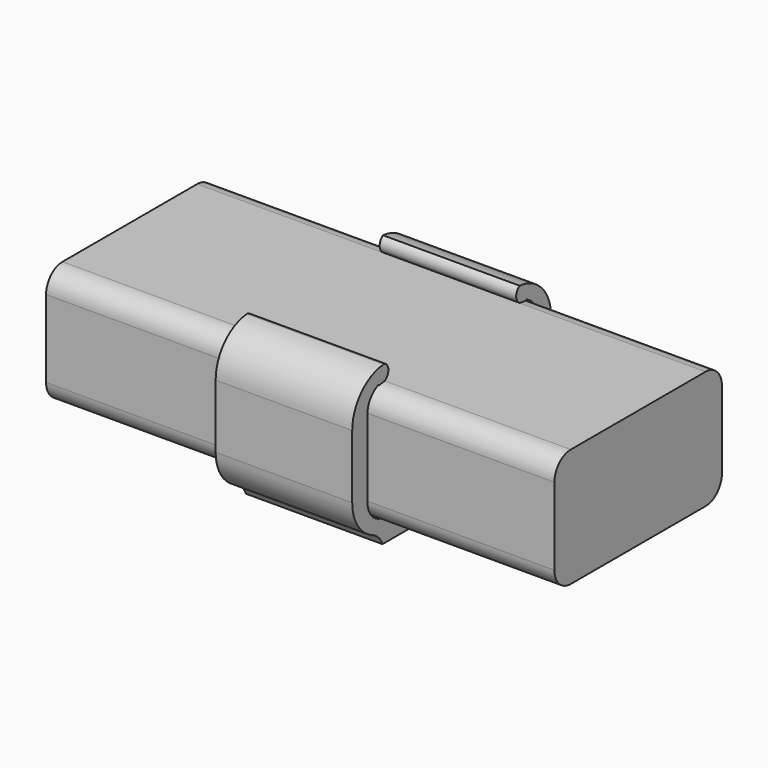
from build123d import *

# Parameters (mm, degrees)
F1_DEPTH       = 55.825
F3_DEPTH       = 15
F5_D           = 6.5
F5_CBORE_D     = 10.6
F5_CBORE_DEPTH = 3.4
F6_T1_DEPTH    = 30
F7_R           = 1


# Not quite as in the source:
# - a fillet or chamfer that OpenCascade refuses, or shapes differently, is made with other operations: its cross-section is extruded or revolved along the edge and cut away or added


with BuildPart() as f1:
    # F0 (on Right) → F1 (new body, symmetric)
    with BuildSketch(Plane.YZ):
        with BuildLine():
            ThreePointArc((-23, 4.5), (-21.6819805153, 1.3180194847), (-18.5, 0))
            Line((-18.5, 0), (18.5, 0))
            ThreePointArc((18.5, 0), (21.6819805153, 1.3180194847), (23, 4.5))
            Line((23, 4.5), (23, 21.5))
            ThreePointArc((23, 21.5), (21.6819805153, 24.6819805153), (18.5, 26))
            Line((18.5, 26), (-18.5, 26))
            ThreePointArc((-18.5, 26), (-21.6819805153, 24.6819805153), (-23, 21.5))
            Line((-23, 21.5), (-23, 4.5))
        make_face()
    extrude(amount=F1_DEPTH, both=True)


with BuildPart() as f3:
    # F2 (on Right) → F3 (new body, symmetric)
    with BuildSketch(Plane.YZ):
        with BuildLine():
            add(Edge.make_bspline(
                [(26.7413663264, 22.9510836938), (26.7479851877, 22.9405500746), (26.746124128, 22.9346023266), (26.7444516472, 22.9402163477)],
                knots=[0.9580519354, 0.9580519354, 0.9580519354, 0.9580519354, 1, 1, 1, 1], degree=3))
            ThreePointArc((26.7413663264, 22.9510836938), (26.7429106369, 22.9456504892), (26.7444516472, 22.9402163477))
        make_face()
    extrude(amount=F3_DEPTH, both=True)


with BuildPart() as f3b:
    # F2 (on Right) → F3, piece 2 (new body, symmetric)
    with BuildSketch(Plane.YZ):
        with BuildLine():
            Line((23.3, 21.5), (23.3, 4.5))
            ThreePointArc((23.3, 4.5), (21.8941125497, 1.1058874503), (18.5, -0.3))
            Line((18.5, -0.3), (-18.5, -0.3))
            ThreePointArc((-18.5, -0.3), (-21.8941125497, 1.1058874503), (-23.3, 4.5))
            Line((-23.3, 4.5), (-23.3, 21.5))
            ThreePointArc((-23.3, 21.5), (-22.4816132456, 24.1808125563), (-20.3055183491, 25.9474828264))
            ThreePointArc((-20.3055183491, 25.9474828264), (-17.7711928448, 26.7933262745), (-18.4856994576, 29.3677654758))
            ThreePointArc((-18.4856994576, 29.3677654758), (-24.8705621503, 26.5239553831), (-27.4715276401, 20.0363744805))
            Line((-27.4715276401, 20.0363744805), (-27.4715276401, 6.0863744805))
            ThreePointArc((-27.4715276401, 6.0863744805), (-25.0921489995, -0.126112944), (-19.1715276401, -3.1597057701))
            Line((-19.1715276401, -3.1597057701), (-19.1715276401, -5.3))
            Line((-19.1715276401, -5.3), (18.7964805483, -5.3))
            Line((18.7964805483, -5.3), (18.7964805483, -2.7903881607))
            ThreePointArc((18.7964805483, -2.7903881607), (24.7171019077, 0.2432046654), (27.0964805483, 6.4556920899))
            Line((27.0964805483, 6.4556920899), (27.0964805483, 20.4056920899))
            ThreePointArc((27.0964805483, 20.4056920899), (26.9504507259, 21.7510160985), (26.6111170191, 23.0610061873))
            add(Edge.make_bspline(
                [(21.8595435659, 24.928332981), (23.3056451816, 24.9760065601), (25.9834803549, 23.5080012929), (26.6111170191, 23.0610061873)],
                knots=[0.1665026568, 0.1665026568, 0.1665026568, 0.1665026568, 0.8763222388, 0.8763222388, 0.8763222388, 0.8763222388], degree=3))
            ThreePointArc((21.8595435659, 24.928332981), (22.9252575697, 23.3593266097), (23.3, 21.5))
        make_face()
        with BuildLine():
            ThreePointArc((20.3055183491, 25.9474828264), (21.1323245903, 25.5138344823), (21.8595435659, 24.928332981))
            add(Edge.make_bspline(
                [(21.8595435659, 24.928332981), (23.3056451816, 24.9760065601), (25.9834803549, 23.5080012929), (26.6111170191, 23.0610061873)],
                knots=[0.1665026568, 0.1665026568, 0.1665026568, 0.1665026568, 0.8763222388, 0.8763222388, 0.8763222388, 0.8763222388], degree=3))
            ThreePointArc((26.6111170191, 23.0610061873), (23.4973497148, 27.4369702659), (18.4856994576, 29.3677654758))
            ThreePointArc((18.4856994576, 29.3677654758), (17.7711928448, 26.7933262745), (20.3055183491, 25.9474828264))
        make_face()
    extrude(amount=F3_DEPTH, both=True)

    # F5 (through all)
    with Locations(Plane.XY.offset(-0.3)):
        with Locations((-8.4035573527, 0), (8.4035573527, 0)):
            CounterBoreHole(F5_D / 2, F5_CBORE_D / 2, F5_CBORE_DEPTH)

    # F6: fillet of radius 5 on 2 edges, made by hand

    # F6_s2 → F6_t1 (join)
    with BuildSketch(Plane.YZ.offset(-15)):
        with BuildLine():
            ThreePointArc((18.7964805483, -5.3), (19.8233418664, -3.3539370541), (21.5861905231, -2.0371341951))
            ThreePointArc((21.5861905231, -2.0371341951), (20.2207697833, -2.522772239), (18.7964805483, -2.7903881607))
            Line((18.7964805483, -2.7903881607), (18.7964805483, -5.3))
        make_face()
        with BuildLine():
            ThreePointArc((-21.8721121654, -2.4456636213), (-20.2296725429, -3.5964212779), (-19.1715276401, -5.3))
            Line((-19.1715276401, -5.3), (-19.1715276401, -3.1597057701))
            ThreePointArc((-19.1715276401, -3.1597057701), (-20.5487818898, -2.9046578425), (-21.8721121654, -2.4456636213))
        make_face()
    extrude(amount=F6_T1_DEPTH)

    # F7
    f7_edges = [f3b.edges().sort_by_distance(p)[0] for p in [
        (0, -18.485699, 29.367765),
    ]]
    fillet(f7_edges, radius=F7_R)


solid = Compound([f1.part, f3.part, f3b.part])
